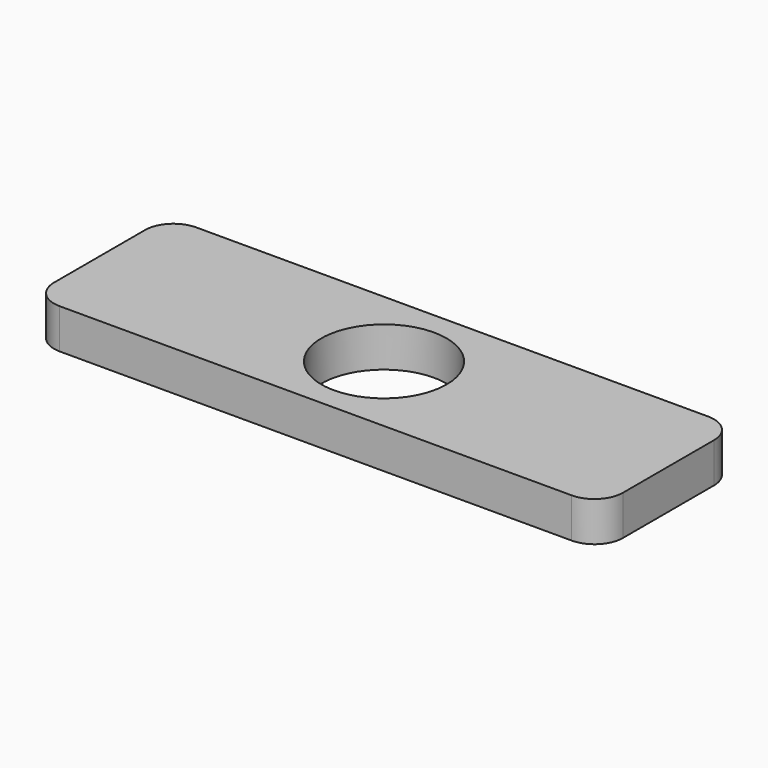
from build123d import *

# Parameters (mm, degrees)
F0_R     = 11
F1_DEPTH = 7


# Not quite as in the source:
# - a feature of the source that left no trace in its solid (it failed there, or was rolled back) is left out


with BuildPart() as f1:
    # F0 (on Top) → F1 (new body)
    with BuildSketch(Plane.XY):
        with BuildLine():
            Line((-45, -15), (45, -15))
            ThreePointArc((45, -15), (48.5355339059, -13.5355339059), (50, -10))
            Line((50, -10), (50, 10))
            ThreePointArc((50, 10), (48.5355339059, 13.5355339059), (45, 15))
            Line((45, 15), (-45, 15))
            ThreePointArc((-45, 15), (-48.5355339059, 13.5355339059), (-50, 10))
            Line((-50, 10), (-50, -10))
            ThreePointArc((-50, -10), (-48.5355339059, -13.5355339059), (-45, -15))
        make_face()
        Circle(F0_R, mode=Mode.SUBTRACT)
    extrude(amount=F1_DEPTH)


solid = f1.part
